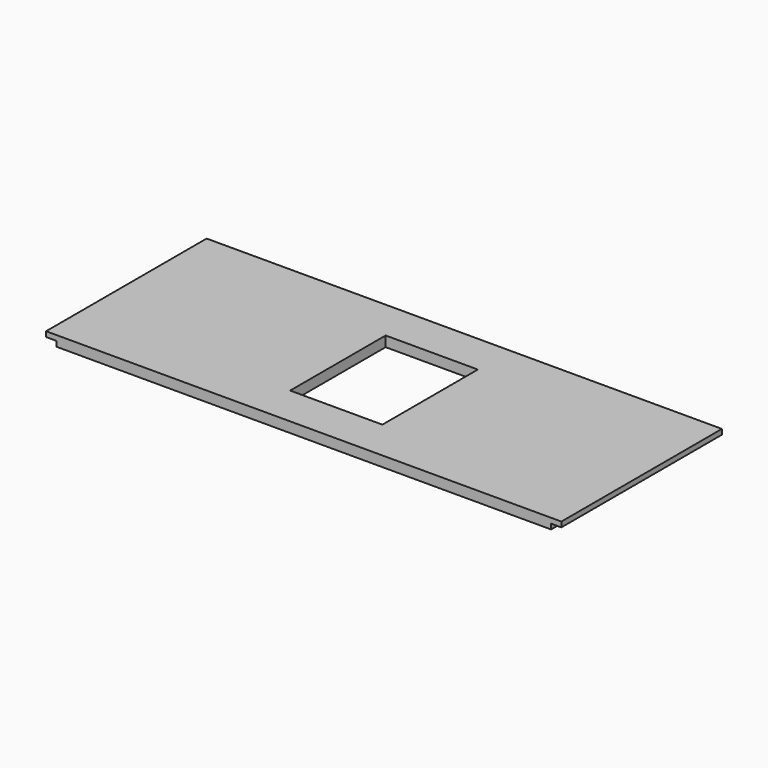
from build123d import *

# Parameters (mm, degrees)
F1_W      = 603.25
F1_H      = 234.95
F2_DEPTH  = 12.065
F3_W      = 12.065
F3_H      = 234.95
F4_DEPTH  = 6.0325
F5_W      = 12.065
F5_H      = 234.95
F6_DEPTH  = 6.0325
F7_W      = 12.065
F7_H      = 234.95
F8_DEPTH  = 6.0325
F9_W      = 12.065
F9_H      = 234.95
F10_DEPTH = 6.0325
F11_W     = 203.2
F11_H     = 12.065
F14_DEPTH = 6.0325
F12_W     = 148.59
F12_H     = 12.065
F15_DEPTH = 6.0325
F13_W     = 203.2
F13_H     = 12.065
F16_DEPTH = 6.0325
F17_W     = 12.065
F17_H     = 31.75
F18_DEPTH = 6.0325
F19_W     = 12.065
F19_H     = 31.75
F20_DEPTH = 6.0325
F21_W     = 107.95
F21_H     = 139.7
F22_DEPTH = 12.065


# Not quite as in the source:
# - a variable given as a bare number and used for a length is read in inches; the dataset says mm whatever the document's units were


with BuildPart() as f2:
    # F1 (on Top) → F2 (new body)
    with BuildSketch(Plane.XY):
        Rectangle(F1_W, F1_H)
    extrude(amount=F2_DEPTH)

    # F3 (on face) → F4 (cut)
    with BuildSketch(Plane(origin=(0, 0, 0), x_dir=(1, 0, 0), z_dir=(0, 0, -1))):
        with Locations((-295.5925, 0)):
            Rectangle(F3_W, F3_H)
    extrude(amount=-F4_DEPTH, mode=Mode.SUBTRACT)

    # F5 (on face) → F6 (cut)
    with BuildSketch(Plane(origin=(0, 0, 0), x_dir=(1, 0, 0), z_dir=(0, 0, -1))):
        with Locations((295.5925, 0)):
            Rectangle(F5_W, F5_H)
    extrude(amount=-F6_DEPTH, mode=Mode.SUBTRACT)

    # F7 (on face) → F8 (cut)
    with BuildSketch(Plane(origin=(0, 0, 0), x_dir=(1, 0, 0), z_dir=(0, 0, -1))):
        with Locations((80.3275, 0)):
            Rectangle(F7_W, F7_H)
    extrude(amount=-F8_DEPTH, mode=Mode.SUBTRACT)

    # F9 (on face) → F10 (cut)
    with BuildSketch(Plane(origin=(0, 0, 0), x_dir=(1, 0, 0), z_dir=(0, 0, -1))):
        with Locations((-80.3275, 0)):
            Rectangle(F9_W, F9_H)
    extrude(amount=-F10_DEPTH, mode=Mode.SUBTRACT)

    # F11 (on face) → F14 (cut)
    with BuildSketch(Plane(origin=(0, 0, 0), x_dir=(1, 0, 0), z_dir=(0, 0, -1))):
        with Locations((187.96, -111.4425)):
            Rectangle(F11_W, F11_H)
    extrude(amount=-F14_DEPTH, mode=Mode.SUBTRACT)

    # F12 (on face) → F15 (cut)
    with BuildSketch(Plane(origin=(0, 0, 0), x_dir=(1, 0, 0), z_dir=(0, 0, -1))):
        with Locations((0, -111.4425)):
            Rectangle(F12_W, F12_H)
    extrude(amount=-F15_DEPTH, mode=Mode.SUBTRACT)

    # F13 (on face) → F16 (cut)
    with BuildSketch(Plane(origin=(0, 0, 0), x_dir=(1, 0, 0), z_dir=(0, 0, -1))):
        with Locations((-187.96, -111.4425)):
            Rectangle(F13_W, F13_H)
    extrude(amount=-F16_DEPTH, mode=Mode.SUBTRACT)

    # F17 (on face) → F18 (join)
    with BuildSketch(Plane(origin=(0, 0, 6.0325), x_dir=(1, 0, 0), z_dir=(0, 0, -1))):
        with Locations((80.3275, 101.6)):
            Rectangle(F17_W, F17_H)
    extrude(amount=F18_DEPTH)

    # F19 (on face) → F20 (join)
    with BuildSketch(Plane(origin=(0, 0, 6.0325), x_dir=(1, 0, 0), z_dir=(0, 0, -1))):
        with Locations((-80.3275, 101.6)):
            Rectangle(F19_W, F19_H)
    extrude(amount=F20_DEPTH)

    # F21 (on face) → F22 (cut)
    with BuildSketch(Plane.XY.offset(12.065)):
        Rectangle(F21_W, F21_H)
    extrude(amount=-F22_DEPTH, mode=Mode.SUBTRACT)


solid = f2.part
